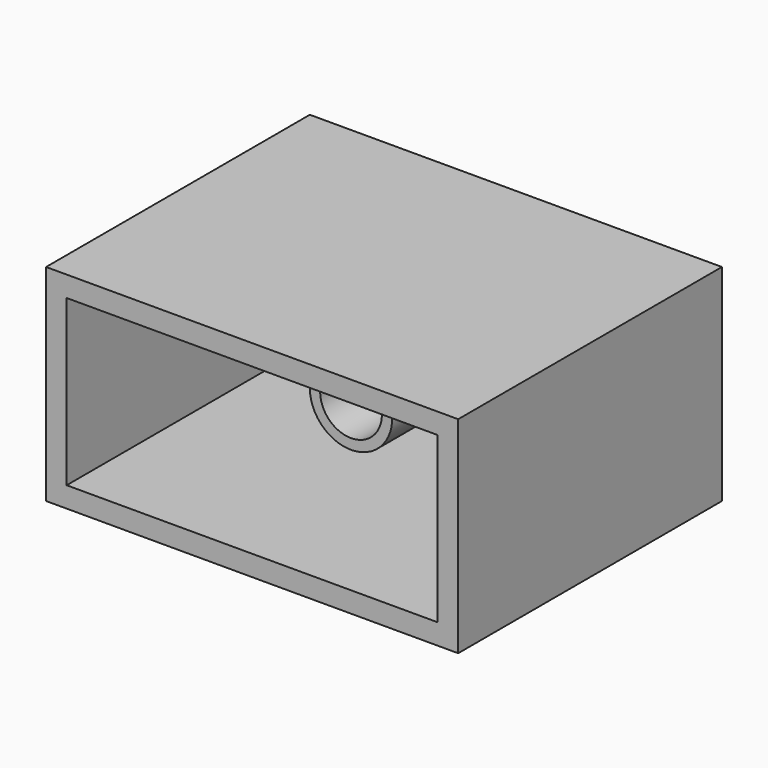
from build123d import *

# Parameters (mm, degrees)
F0_W        = 100
F0_H        = 50
F1_DEPTH    = 80
F2_T        = -5
F3_R        = 10
F4_DEPTH    = 50
F5_T        = 2.5
F5_T3_DEPTH = 80
F5_T5_DEPTH = 45
F5_T7_DEPTH = 95


# Not quite as in the source:
# - a shell that OpenCascade refuses in one call is made with other operations: the cavity is built on its own and cut out


with BuildPart() as f1:
    # F0 (on Front) → F1 (new body)
    with BuildSketch(Plane.XZ):
        Rectangle(F0_W, F0_H)
    extrude(amount=F1_DEPTH)

    # F2
    f2_openings = [f1.faces().sort_by_distance(p)[0] for p in [
        (0, -80, 0),
    ]]
    offset(amount=F2_T, openings=f2_openings)

    # F3 (on face) → F4 (join)
    with BuildSketch(Plane(origin=(0, 0, 0), x_dir=(-1, 0, 0), z_dir=(0, 1, 0))):
        Circle(F3_R)
    extrude(amount=-F4_DEPTH)

    # F5: shell of thickness 2.5, made by hand


with BuildPart() as f5_core1:
    # F5_t2: copy of F1
    add(f1.part)

    # the walls: a layer under each face that stays
    f5_faces = [f5_core1.faces().sort_by_distance(p)[0] for p in [
        (-50, -40, 0),
        (0, -40, 25),
        (0, -40, -25),
        (0, 0, 0),
        (-42.8571428571, -80, -21.4285714286),
        (50, -40, 0),
        (-45, -42.5, 0),
        (0, -42.5, 20),
        (45, -42.5, 0),
        (0, -42.5, -20),
        (-30, -5, -13.3333333333),
        (10, -27.5, 0),
    ]]
    thicken(f5_faces, amount=-F5_T, mode=Mode.SUBTRACT)

    # F5_s4 → F5_t3 (cut)
    with BuildSketch(Plane.XZ.offset(2.5)):
        Polygon((-44.975, -19.975), (-47.5, -20), (-47.5, -22.5), (-45, -22.5), align=None)
        Polygon((-44.975, 19.975), (-47.5, 20), (-47.5, 22.5), (-45, 22.5), align=None)
        Polygon((44.975, 19.975), (45, 22.5), (47.5, 22.5), (47.5, 20), align=None)
        Polygon((44.975, -19.975), (47.5, -20), (47.5, -22.5), (45, -22.5), align=None)
    extrude(amount=F5_T3_DEPTH, mode=Mode.SUBTRACT)

    # F5_s6 → F5_t5 (cut)
    with BuildSketch(Plane.XY.offset(-22.5)):
        Polygon((-44.975, -5.025), (-47.5, -5), (-47.5, -2.5), (-45, -2.5), align=None)
        Polygon((44.975, -5.025), (47.5, -5), (47.5, -2.5), (45, -2.5), align=None)
    extrude(amount=F5_T5_DEPTH, mode=Mode.SUBTRACT)

    # F5_s8 → F5_t7 (cut)
    with BuildSketch(Plane.YZ.offset(-47.5)):
        Polygon((-5.025, 19.975), (-5, 22.5), (-2.5, 22.5), (-2.5, 20), align=None)
        Polygon((-5.025, -19.975), (-5, -22.5), (-2.5, -22.5), (-2.5, -20), align=None)
    extrude(amount=F5_T7_DEPTH, mode=Mode.SUBTRACT)

    # F5_s9 → F5_t10 (revolve, cut)
    with BuildSketch(Plane.XY):
        Polygon((-10.025, -5.025), (-10, -2.5), (-7.5, -2.5), (-7.5, -5), align=None)
    revolve(axis=Axis((0, -5, 0), (0, 1, 0)), mode=Mode.SUBTRACT)


with BuildPart() as f1_1:
    add(f1.part)

    # what is left inside the walls is the cavity
    f5_cavity = [f5_core1.part.solids().sort_by_distance(p)[0] for p in [
        (7.475, -18.333333, 0),
    ]]
    add(f5_cavity, mode=Mode.SUBTRACT)


solid = f1_1.part
